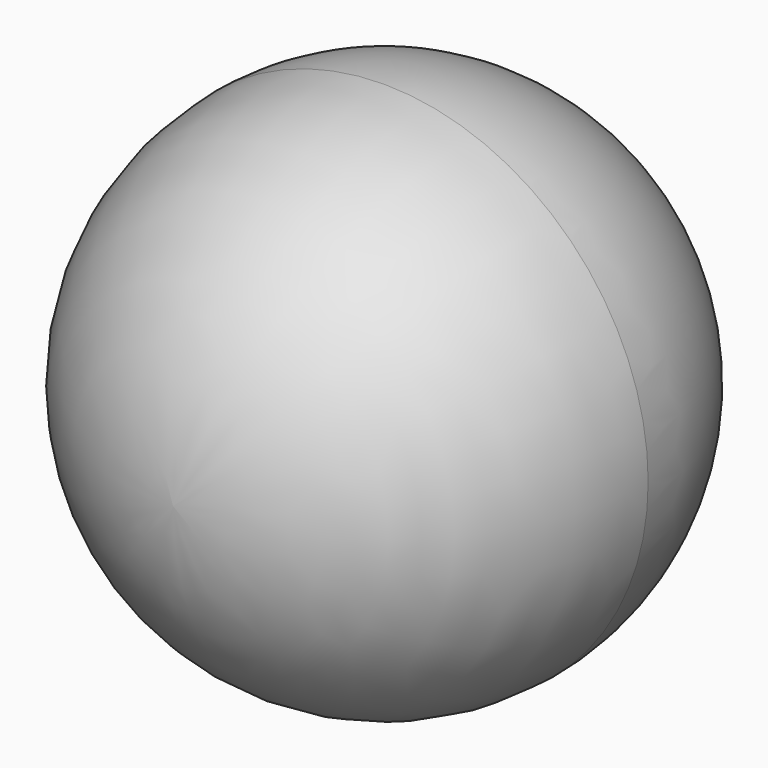
from build123d import *

# Parameters (mm, degrees)
F0_R     = 50.8
F1_DEPTH = 50.8
F2_R     = 50.79999


# Not quite as in the source:
# - a fillet or chamfer is up to 0.001 mm smaller than in the source, because OpenCascade refuses the exact size


with BuildPart() as f1:
    # F0 (on Front) → F1 (new body)
    with BuildSketch(Plane.XZ):
        Circle(F0_R)
    extrude(amount=F1_DEPTH)

    # F2 (radius 50.8 in the source; OpenCascade refuses exactly that, so slightly less here)
    f2_edges = [f1.edges().sort_by_distance(p)[0] for p in [
        (-50.8, -50.8, 0),
    ]]
    fillet(f2_edges, radius=F2_R)

    # F3 (on Front) → F4 (revolve)
    with BuildSketch(Plane.XZ):
        with BuildLine():
            ThreePointArc((0, -50.8), (50.8, 0), (0, 50.8))
            Line((0, 50.8), (0, -50.8))
        make_face()
    revolve(axis=Axis((0, 0, 0.4323792445), (0, 0, -1)))


solid = f1.part
